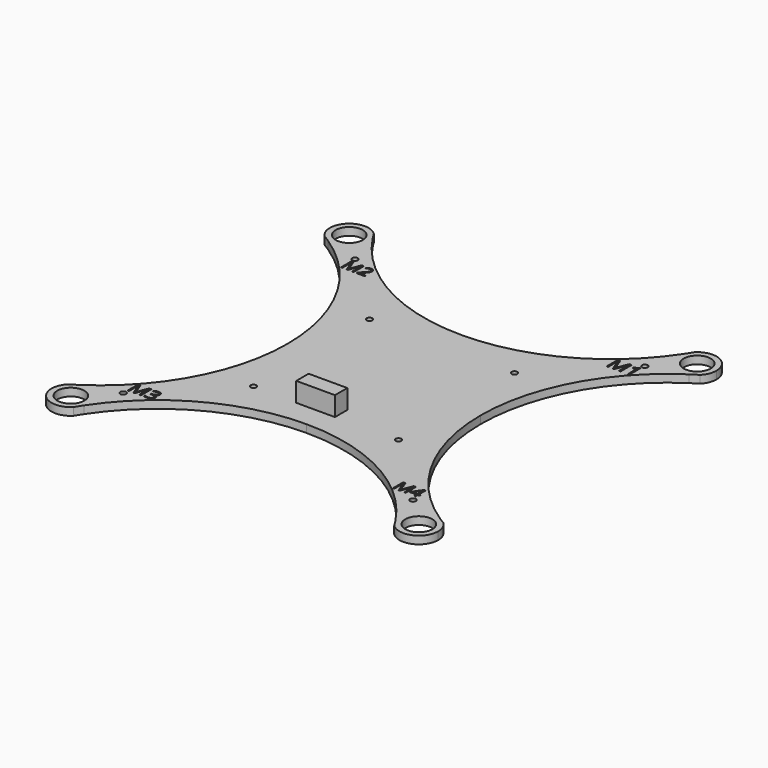
from build123d import *

# Parameters (mm, degrees)
F0_R           = 0.75
F0_R_2         = 3.5
F1_DEPTH       = 2
F2_W           = 10
F2_H           = 4
F3_DEPTH       = 5
F4_TEXT_SIZE   = 4.8290452637
F4_TEXT_SIZE_2 = 4.6405391738
F4_TEXT_SIZE_3 = 5.0707311463
F4_TEXT_SIZE_4 = 4.672013601
F5_DEPTH       = 25


# Not quite as in the source:
# - Text() gives the source's letters only with a copy of the font that has no kerning and outlines rounded to 1/6400 em; it was checked with that copy


with BuildPart() as f1:
    # F0 (on Top) → F1 (new body)
    with BuildSketch(Plane.XY):
        with BuildLine():
            ThreePointArc((40.2815340503, 46.6541097549), (22.8664735733, 30.7566251819), (0, 25))
            ThreePointArc((0, 25), (-22.8664735733, 30.7566251819), (-40.2815340503, 46.6541097549))
            ThreePointArc((-40.2815340503, 46.6541097549), (-40.070885995, 45.8389488218), (-40, 45))
            ThreePointArc((-40, 45), (-42.1078164628, 40.9213636608), (-46.6541097549, 40.2815340503))
            ThreePointArc((-46.6541097549, 40.2815340503), (-30.7566251819, 22.8664735733), (-25, 0))
            ThreePointArc((-25, 0), (-30.7566251819, -22.8664735733), (-46.6541097549, -40.2815340503))
            ThreePointArc((-46.6541097549, -40.2815340503), (-42.1078164628, -40.9213636608), (-40, -45))
            ThreePointArc((-40, -45), (-40.070885995, -45.8389488218), (-40.2815340503, -46.6541097549))
            ThreePointArc((-40.2815340503, -46.6541097549), (-22.8664735733, -30.7566251819), (0, -25))
            ThreePointArc((0, -25), (22.8664735733, -30.7566251819), (40.2815340503, -46.6541097549))
            ThreePointArc((40.2815340503, -46.6541097549), (41.4644660941, -41.4644660941), (46.6541097549, -40.2815340503))
            ThreePointArc((46.6541097549, -40.2815340503), (30.7566251819, -22.8664735733), (25, 0))
            ThreePointArc((25, 0), (30.7566251819, 22.8664735733), (46.6541097549, 40.2815340503))
            ThreePointArc((46.6541097549, 40.2815340503), (41.4644660941, 41.4644660941), (40.2815340503, 46.6541097549))
        make_face()
        with Locations((-37.4766594029, -37.4766594029)):
            Circle(F0_R, mode=Mode.SUBTRACT)
        with Locations((-18.75, -18.75)):
            Circle(F0_R, mode=Mode.SUBTRACT)
        with Locations((37.4766594029, -37.4766594029)):
            Circle(F0_R, mode=Mode.SUBTRACT)
        with Locations((18.75, -18.75)):
            Circle(F0_R, mode=Mode.SUBTRACT)
        with Locations((-18.75, 18.75)):
            Circle(F0_R, mode=Mode.SUBTRACT)
        with Locations((-37.4766594029, 37.4766594029)):
            Circle(F0_R, mode=Mode.SUBTRACT)
        with Locations((18.75, 18.75)):
            Circle(F0_R, mode=Mode.SUBTRACT)
        with Locations((37.4766594029, 37.4766594029)):
            Circle(F0_R, mode=Mode.SUBTRACT)
        with BuildLine():
            ThreePointArc((-40, -45), (-42.1078164628, -40.9213636608), (-46.6541097549, -40.2815340503))
            ThreePointArc((-46.6541097549, -40.2815340503), (-47.5880162917, -40.8838241131), (-48.5355339059, -41.4644660941))
            ThreePointArc((-48.5355339059, -41.4644660941), (-48.5355339059, -48.5355339059), (-41.4644660941, -48.5355339059))
            ThreePointArc((-41.4644660941, -48.5355339059), (-40.8838241131, -47.5880162917), (-40.2815340503, -46.6541097549))
            ThreePointArc((-40.2815340503, -46.6541097549), (-40.070885995, -45.8389488218), (-40, -45))
        make_face()
        with Locations((-45, -45)):
            Circle(F0_R_2, mode=Mode.SUBTRACT)
        with BuildLine():
            ThreePointArc((48.5355339059, -41.4644660941), (47.5880162917, -40.8838241131), (46.6541097549, -40.2815340503))
            ThreePointArc((46.6541097549, -40.2815340503), (41.4644660941, -41.4644660941), (40.2815340503, -46.6541097549))
            ThreePointArc((40.2815340503, -46.6541097549), (40.8838241131, -47.5880162917), (41.4644660941, -48.5355339059))
            ThreePointArc((41.4644660941, -48.5355339059), (46.9134171618, -49.6193976626), (50, -45))
            ThreePointArc((50, -45), (49.6193976626, -43.0865828382), (48.5355339059, -41.4644660941))
        make_face()
        with Locations((45, -45)):
            Circle(F0_R_2, mode=Mode.SUBTRACT)
        with BuildLine():
            ThreePointArc((41.4644660941, 48.5355339059), (40.8838241131, 47.5880162917), (40.2815340503, 46.6541097549))
            ThreePointArc((40.2815340503, 46.6541097549), (41.4644660941, 41.4644660941), (46.6541097549, 40.2815340503))
            ThreePointArc((46.6541097549, 40.2815340503), (47.5880162917, 40.8838241131), (48.5355339059, 41.4644660941))
            ThreePointArc((48.5355339059, 41.4644660941), (49.6193976626, 43.0865828382), (50, 45))
            ThreePointArc((50, 45), (46.9134171618, 49.6193976626), (41.4644660941, 48.5355339059))
        make_face()
        with Locations((45, 45)):
            Circle(F0_R_2, mode=Mode.SUBTRACT)
        with BuildLine():
            ThreePointArc((-40, 45), (-40.070885995, 45.8389488218), (-40.2815340503, 46.6541097549))
            ThreePointArc((-40.2815340503, 46.6541097549), (-40.8838241131, 47.5880162917), (-41.4644660941, 48.5355339059))
            ThreePointArc((-41.4644660941, 48.5355339059), (-48.5355339059, 48.5355339059), (-48.5355339059, 41.4644660941))
            ThreePointArc((-48.5355339059, 41.4644660941), (-47.5880162917, 40.8838241131), (-46.6541097549, 40.2815340503))
            ThreePointArc((-46.6541097549, 40.2815340503), (-42.1078164628, 40.9213636608), (-40, 45))
        make_face()
        with Locations((-45, 45)):
            Circle(F0_R_2, mode=Mode.SUBTRACT)
    extrude(amount=F1_DEPTH)

    # F2 (on face) → F3 (join)
    with BuildSketch(Plane.XY.offset(2)):
        with Locations((-2.5, -17)):
            Rectangle(F2_W, F2_H)
    extrude(amount=F3_DEPTH)

    # F4 (on face) → F5 (cut)
    with BuildSketch(Plane.XY.offset(2)):
        with Locations((-37.9319396766, -36.0808738818)):
            Text('M3', F4_TEXT_SIZE, font='Open Sans', text_align=(TextAlign.LEFT, TextAlign.BOTTOM))
        with Locations((30.6163570378, -35.945149497)):
            Text('M4', F4_TEXT_SIZE_2, font='Open Sans', text_align=(TextAlign.LEFT, TextAlign.BOTTOM))
        with Locations((30.9903494685, 32.6039612919)):
            Text('M1', F4_TEXT_SIZE_3, font='Open Sans', text_align=(TextAlign.LEFT, TextAlign.BOTTOM))
        with Locations((-37.9319396766, 32.8910379245)):
            Text('M2', F4_TEXT_SIZE_4, font='Open Sans', text_align=(TextAlign.LEFT, TextAlign.BOTTOM))
    extrude(amount=-F5_DEPTH, mode=Mode.SUBTRACT)


solid = f1.part
